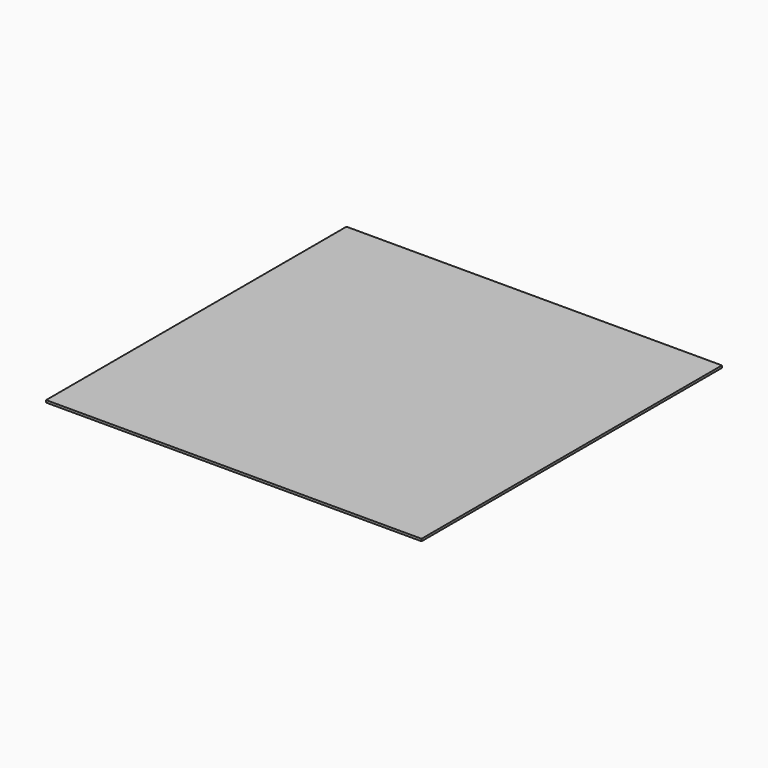
from build123d import *

# Parameters (mm, degrees)
F1_W     = 500
F1_H     = 500
F2_DEPTH = 3


with BuildPart() as f2:
    # F1 (on Top) → F2 (new body)
    with BuildSketch(Plane.XY):
        Rectangle(F1_W, F1_H)
    extrude(amount=F2_DEPTH)


solid = f2.part
